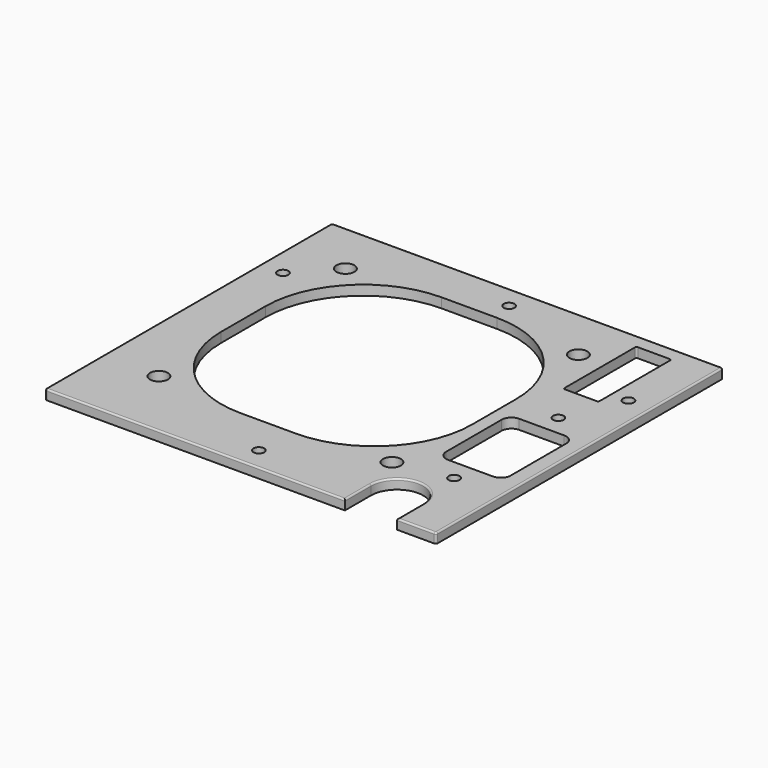
from build123d import *

# Parameters (mm, degrees)
F1_DEPTH  = 3
F3_D      = 3.3
F5_D      = 5.5
F6_DEPTH  = 3.001
F7_R      = 0.6
F8_R      = 0.5
F10_D     = 3.3
F11_DEPTH = 3.001
F12_W     = 10.8
F12_H     = 28
F13_DEPTH = 3.001
F14_R     = 0.5


# Not quite as in the source:
# - a feature names something its author has since deleted; it is built from what else it names


with BuildPart() as f1:
    # F0 (on Top) → F1 (new body)
    with BuildSketch(Plane.XY):
        with BuildLine():
            Line((60, 55), (-60, 55))
            Line((-60, 55), (-60, -55))
            Line((-60, -55), (32, -55))
            Line((32, -55), (32, -45))
            ThreePointArc((32, -45), (40, -37), (48, -45))
            Line((48, -45), (48, -55))
            Line((48, -55), (60, -55))
            Line((60, -55), (60, 55))
        make_face()
    extrude(amount=F1_DEPTH)

    # F3 (through all)
    with Locations(Plane.XY.offset(3)):
        with Locations((-53, 27.5), (0, 48), (53, 27.5), (0, -48)):
            Hole(F3_D / 2)

    # F5 (through all)
    with Locations(Plane.XY.offset(3)):
        with Locations((-42.7202362838, 38.5875506155), (-42.7202362838, -32.9124493845), (28.7797637162, -32.9124493845), (28.7797637162, 38.5875506155)):
            Hole(F5_D / 2)

    # F4 (on face) → F6 (cut, through all)
    with BuildSketch(Plane.XY.offset(3)):
        with BuildLine():
            ThreePointArc((31.5297637162, 11.3375506155), (22.7429671518, 32.5507540511), (1.5297637162, 41.3375506155))
            Line((1.5297637162, 41.3375506155), (-15.4702362838, 41.3375506155))
            ThreePointArc((-15.4702362838, 41.3375506155), (-36.6834397194, 32.5507540511), (-45.4702362838, 11.3375506155))
            Line((-45.4702362838, 11.3375506155), (-45.4702362838, -5.6624493845))
            ThreePointArc((-45.4702362838, -5.6624493845), (-36.6834397194, -26.8756528201), (-15.4702362838, -35.6624493845))
            Line((-15.4702362838, -35.6624493845), (1.5297637162, -35.6624493845))
            ThreePointArc((1.5297637162, -35.6624493845), (22.7429671518, -26.8756528201), (31.5297637162, -5.6624493845))
            Line((31.5297637162, -5.6624493845), (31.5297637162, 11.3375506155))
        make_face()
    extrude(amount=-F6_DEPTH, mode=Mode.SUBTRACT)

    # F7
    f7_edges = [f1.edges().sort_by_distance(p)[0] for p in [
        (-60, 55, 1.5),
        (60, 55, 1.5),
        (60, -55, 1.5),
        (-60, -55, 1.5),
    ]]
    fillet(f7_edges, radius=F7_R)

    # F8
    f8_edges = [f1.edges().sort_by_distance(p)[0] for p in [
        (40, -37, 3),
        (-13.7, -55, 3),
    ]]
    fillet(f8_edges, radius=F8_R)

    # F10 (through all)
    with Locations(Plane.XY.offset(3)):
        with Locations((45.5, 10), (45.5, -30)):
            Hole(F10_D / 2)

    # F9 (on face) → F11 (cut, through all)
    with BuildSketch(Plane.XY.offset(3)):
        with BuildLine():
            Line((52.3, 3.75), (38.5, 3.75))
            ThreePointArc((38.5, 3.75), (36.3786796564, 2.8713203436), (35.5, 0.75))
            Line((35.5, 0.75), (35.5, -20.55))
            ThreePointArc((35.5, -20.55), (36.3786796564, -22.6713203436), (38.5, -23.55))
            Line((38.5, -23.55), (52.3, -23.55))
            ThreePointArc((52.3, -23.55), (54.4213203436, -22.6713203436), (55.3, -20.55))
            Line((55.3, -20.55), (55.3, 0.75))
            ThreePointArc((55.3, 0.75), (54.4213203436, 2.8713203436), (52.3, 3.75))
        make_face()
    extrude(amount=-F11_DEPTH, mode=Mode.SUBTRACT)

    # F12 (on face) → F13 (cut, through all)
    with BuildSketch(Plane.XY.offset(3)):
        with Locations((42.4, 36.5)):
            Rectangle(F12_W, F12_H)
    extrude(amount=-F13_DEPTH, mode=Mode.SUBTRACT)

    # F14
    f14_edges = [f1.edges().sort_by_distance(p)[0] for p in [
        (37, 22.5, 1.5),
        (37, 50.5, 1.5),
        (47.8, 50.5, 1.5),
        (47.8, 22.5, 1.5),
    ]]
    fillet(f14_edges, radius=F14_R)


solid = f1.part
